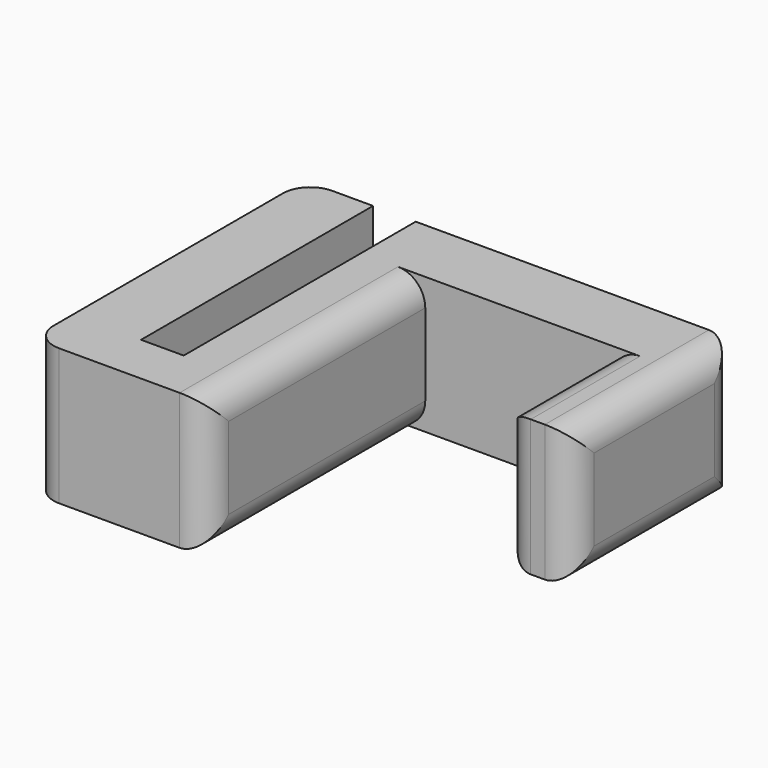
from build123d import *

# Parameters (mm, degrees)
F1_DEPTH     = 25.4
F2_R         = 5.08
F3_TEXT_SIZE = 19.772476258
F4_DEPTH     = 3


# Not quite as in the source:
# - Text() gives the source's letters only with a copy of the font that has no kerning and outlines rounded to 1/6400 em; it was checked with that copy


with BuildPart() as f1:
    # F0 (on Top) → F1 (new body)
    with BuildSketch(Plane.XY):
        Polygon((0, 63.5), (0, 0), (32.5752518936, 0), (32.5752518936, 50.8), (67.4797778515, 50.8), (67.4797778515, 25.3516854542), (80.2734648196, 25.3516854542), (80.2734648196, 63.5), (20.6375, 63.5), (20.6375, 9.52754), (12.7, 9.52754), (12.7, 63.5), align=None)
    extrude(amount=F1_DEPTH)

    # F2
    f2_edges = [f1.edges().sort_by_distance(p)[0] for p in [
        (80.273465, 63.5, 12.7),
        (80.273465, 25.351685, 12.7),
        (67.479778, 25.351685, 12.7),
        (32.575252, 0, 12.7),
        (0, 0, 12.7),
        (0, 63.5, 12.7),
        (32.575252, 25.4, 25.4),
        (67.479778, 38.075843, 25.4),
        (80.273465, 44.425843, 25.4),
        (80.273465, 44.425843, 0),
        (67.479778, 38.075843, 0),
        (32.575252, 25.4, 0),
    ]]
    fillet(f2_edges, radius=F2_R)

    # F3 (on face) → F4 (join)
    with BuildSketch(Plane(origin=(0, 0, 0), x_dir=(0, -1, 0), z_dir=(-1, 0, 0))):
        with Locations((-55.9856947511, 5.5073467083)):
            Text('CALL', F3_TEXT_SIZE, font='Open Sans', font_style=FontStyle.BOLD, text_align=(TextAlign.LEFT, TextAlign.BOTTOM))
    extrude(amount=F4_DEPTH)


solid = f1.part
